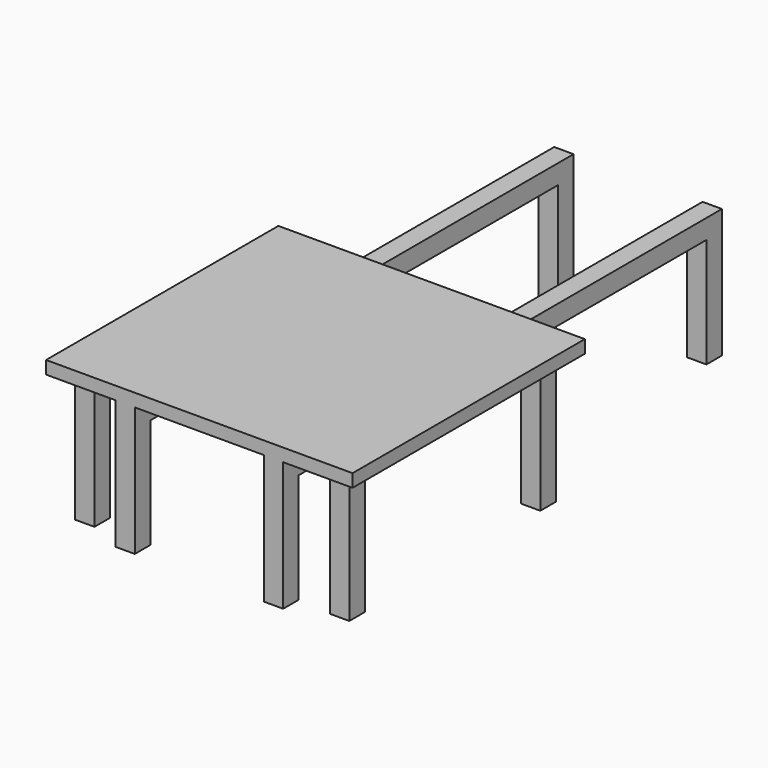
from build123d import *

# Parameters (mm, degrees)
F0_W     = 950
F0_H     = 900
F0_W_2   = 60
F0_H_2   = 60
F1_DEPTH = 40
F2_DEPTH = 400
F3_W     = 60
F3_H     = 1700
F4_DEPTH = 60
F5_DEPTH = 60
F6_W     = 60
F6_H     = 60
F7_DEPTH = 340


# Not quite as in the source:
# - a feature names something its author has since deleted; it is built from what else it names


with BuildPart() as f1:
    # F0 (on Top) → F1 (new body)
    with BuildSketch(Plane.XY):
        with Locations((0, 450)):
            Rectangle(F0_W, F0_H)
        with Locations((-395, 80)):
            Rectangle(F0_W_2, F0_H_2, mode=Mode.SUBTRACT)
        with Locations((395, 80)):
            Rectangle(F0_W_2, F0_H_2, mode=Mode.SUBTRACT)
        with Locations((-395, 820)):
            Rectangle(F0_W_2, F0_H_2, mode=Mode.SUBTRACT)
        with Locations((395, 820)):
            Rectangle(F0_W_2, F0_H_2, mode=Mode.SUBTRACT)
        with Locations((-395, 80)):
            Rectangle(F0_W_2, F0_H_2)
        with Locations((-395, 820)):
            Rectangle(F0_W_2, F0_H_2)
        with Locations((395, 80)):
            Rectangle(F0_W_2, F0_H_2)
        with Locations((395, 820)):
            Rectangle(F0_W_2, F0_H_2)
    extrude(amount=F1_DEPTH)

    # F0 (on Top) → F2 (join)
    with BuildSketch(Plane.XY):
        with Locations((-395, 80)):
            Rectangle(F0_W_2, F0_H_2)
        with Locations((-395, 820)):
            Rectangle(F0_W_2, F0_H_2)
        with Locations((395, 80)):
            Rectangle(F0_W_2, F0_H_2)
        with Locations((395, 820)):
            Rectangle(F0_W_2, F0_H_2)
    extrude(amount=-F2_DEPTH)

    # F3 (on face) → F4 (join)
    with BuildSketch(Plane(origin=(0, 0, 0), x_dir=(1, 0, 0), z_dir=(0, 0, -1))):
        with Locations((-230, -850)):
            Rectangle(F3_W, F3_H)
        with Locations((230, -850)):
            Rectangle(F3_W, F3_H)
    extrude(amount=F4_DEPTH)

    # F3 (on face) → F5 (join)
    with BuildSketch(Plane(origin=(0, 0, 0), x_dir=(1, 0, 0), z_dir=(0, 0, -1))):
        with Locations((-230, -850)):
            Rectangle(F3_W, F3_H)
        with Locations((230, -850)):
            Rectangle(F3_W, F3_H)
    extrude(amount=F5_DEPTH)

    # F6 (on face) → F7 (join)
    with BuildSketch(Plane(origin=(0, 0, -60), x_dir=(1, 0, 0), z_dir=(0, 0, -1))):
        with Locations((230, -1670)):
            Rectangle(F6_W, F6_H)
        with Locations((-230, -1670)):
            Rectangle(F6_W, F6_H)
        with Locations((-230, -30)):
            Rectangle(F6_W, F6_H)
        with Locations((230, -30)):
            Rectangle(F6_W, F6_H)
    extrude(amount=F7_DEPTH)


solid = f1.part
